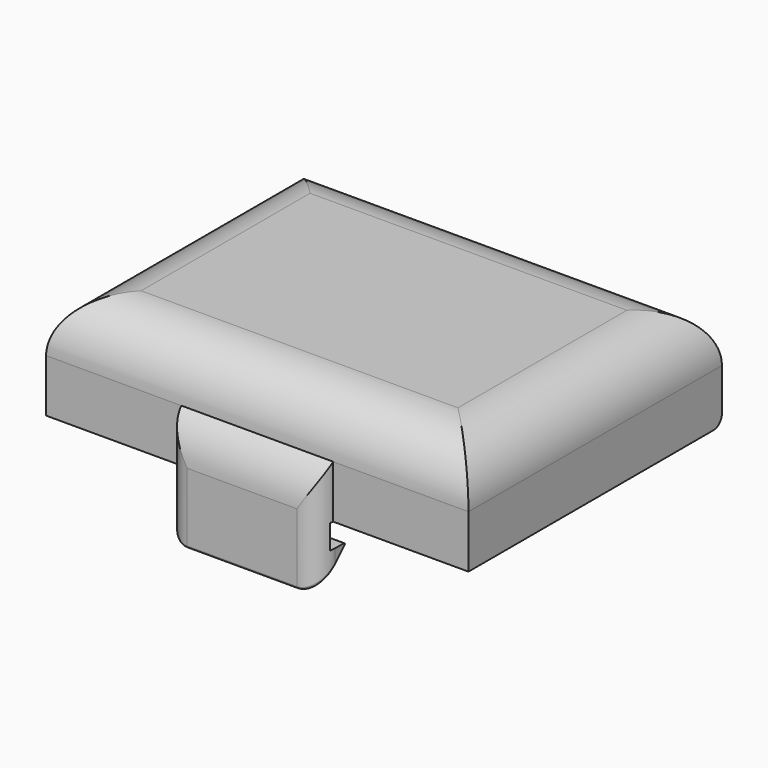
from build123d import *

# Parameters (mm, degrees)
F0_W          = 40
F0_H          = 30
F1_DEPTH      = 10
F2_R          = 5
F3_T          = -3
F4_W          = 27.6
F4_H          = 3
F5_DEPTH      = 3
F6_W          = 46.0305325687
F6_H          = 69.5610698313
F7_DEPTH      = 12.5
F8_R          = 0.55
F9_DEPTH      = 0.55
F10_R         = 0.54999
F11_R         = 1
F13_W         = 14.4
F13_H         = 12
F14_DEPTH     = 1.8
F16_DEPTH     = 25
F17_T4_DEPTH  = 20.8
F17_T9_DEPTH  = 20.8
F17_T14_DEPTH = 20.8
F17_T19_DEPTH = 20.8
F18_T1_DEPTH  = 29.6093727123
F19_R         = 0.2


# Not quite as in the source:
# - a fillet or chamfer that OpenCascade refuses, or shapes differently, is made with other operations: its cross-section is extruded or revolved along the edge and cut away or added
# - a fillet or chamfer is up to 0.001 mm smaller than in the source, because OpenCascade refuses the exact size


with BuildPart() as f1:
    # F0 (on Top) → F1 (new body)
    with BuildSketch(Plane.XY):
        Rectangle(F0_W, F0_H)
    extrude(amount=F1_DEPTH)

    # F2
    f2_edges = [f1.edges().sort_by_distance(p)[0] for p in [
        (20, 0, 10),
        (0, 15, 10),
        (-20, 0, 10),
        (0, -15, 10),
    ]]
    fillet(f2_edges, radius=F2_R)

    # F3
    f3_openings = [f1.faces().sort_by_distance(p)[0] for p in [
        (0, 0, 0),
    ]]
    offset(amount=F3_T, openings=f3_openings)

    # F4 (on Top) → F5 (join)
    with BuildSketch(Plane.XY):
        with Locations((0, 13.5)):
            Rectangle(F4_W, F4_H)
    extrude(amount=-F5_DEPTH)

    # F6 (on Top) → F7 (cut, symmetric)
    with BuildSketch(Plane.XY):
        with Locations((23.0152662843, -8.845419623)):
            Rectangle(F6_W, F6_H)
    extrude(amount=F7_DEPTH, both=True, mode=Mode.SUBTRACT)

    # F8 (on face) → F9 (join)
    with BuildSketch(Plane(origin=(-13.8, 0, 0), x_dir=(0, -1, 0), z_dir=(-1, 0, 0))):
        with Locations((-13.5, -1.5)):
            Circle(F8_R)
    extrude(amount=F9_DEPTH)

    # F10 (radius 0.55 in the source; OpenCascade refuses exactly that, so slightly less here)
    f10_edges = [f1.edges().sort_by_distance(p)[0] for p in [
        (-14.35, 14.05, -1.5),
    ]]
    fillet(f10_edges, radius=F10_R)

    # F11
    f11_edges = [f1.edges().sort_by_distance(p)[0] for p in [
        (-6.9, 15, -3),
        (-6.9, 12, -3),
        (-16.9, 15, 0),
        (-15.4, 12, 0),
    ]]
    fillet(f11_edges, radius=F11_R)

    # F12: F1 across plane


with BuildPart() as f1_1:
    add(f1.part)
    add(f1.part.mirror(Plane.YZ))

    # F13 (on face) → F14 (join, symmetric)
    with BuildSketch(Plane.XZ.offset(15)):
        with Locations((0, -1)):
            Rectangle(F13_W, F13_H)
    extrude(amount=F14_DEPTH, both=True)

    # F15 (on face) → F16 (cut)
    with BuildSketch(Plane(origin=(-7.2, 0, 0), x_dir=(0, -1, 0), z_dir=(-1, 0, 0))):
        Polygon((15.3, 0), (15, 0), (13.2, 0), (13.2, -7), (16.8, -7), (16.8, -5.8), (13.3, -2.3), (15.3, -2.3), align=None)
    extrude(amount=-F16_DEPTH, mode=Mode.SUBTRACT)

    # F17: fillet of radius 2 on 2 edges, made by hand


with BuildPart() as f17_tool2:
    # F17_s3 → F17_t4 (new body)
    with BuildSketch(Plane.XY.offset(10)):
        with BuildLine():
            ThreePointArc((-5.2, -16.8), (-6.6142135624, -16.2142135624), (-7.2, -14.8))
            Line((-7.2, -14.8), (-7.2, -16.8))
            Line((-7.2, -16.8), (-5.2, -16.8))
        make_face()
    extrude(amount=-F17_T4_DEPTH)

    split(bisect_by=Plane.XZ.offset(15), keep=Keep.TOP)


with BuildPart() as f1_2:
    add(f1_1.part)

    # F17_t1: cut F17_tool2
    add(f17_tool2.part, mode=Mode.SUBTRACT)


with BuildPart() as f17_tool7:
    # F17_s8 → F17_t9 (new body)
    with BuildSketch(Plane.XY.offset(10)):
        with BuildLine():
            ThreePointArc((-5.2, -16.8), (-6.6142135624, -16.2142135624), (-7.2, -14.8))
            Line((-7.2, -14.8), (-7.2, -16.8))
            Line((-7.2, -16.8), (-5.2, -16.8))
        make_face()
    extrude(amount=-F17_T9_DEPTH)

    split(bisect_by=Plane.XY, keep=Keep.BOTTOM)


with BuildPart() as f1_3:
    add(f1_2.part)

    # F17_t6: cut F17_tool7
    add(f17_tool7.part, mode=Mode.SUBTRACT)


with BuildPart() as f17_tool12:
    # F17_s13 → F17_t14 (new body)
    with BuildSketch(Plane.XY.offset(-10.8)):
        with BuildLine():
            ThreePointArc((5.2, -16.8), (6.6142135624, -16.2142135624), (7.2, -14.8))
            Line((7.2, -14.8), (7.2, -16.8))
            Line((7.2, -16.8), (5.2, -16.8))
        make_face()
    extrude(amount=F17_T14_DEPTH)

    split(bisect_by=Plane.XZ.offset(15), keep=Keep.TOP)


with BuildPart() as f1_4:
    add(f1_3.part)

    # F17_t11: cut F17_tool12
    add(f17_tool12.part, mode=Mode.SUBTRACT)


with BuildPart() as f17_tool17:
    # F17_s18 → F17_t19 (new body)
    with BuildSketch(Plane.XY.offset(-10.8)):
        with BuildLine():
            ThreePointArc((5.2, -16.8), (6.6142135624, -16.2142135624), (7.2, -14.8))
            Line((7.2, -14.8), (7.2, -16.8))
            Line((7.2, -16.8), (5.2, -16.8))
        make_face()
    extrude(amount=F17_T19_DEPTH)

    split(bisect_by=Plane.XY, keep=Keep.BOTTOM)


with BuildPart() as f1_5:
    add(f1_4.part)

    # F17_t16: cut F17_tool17
    add(f17_tool17.part, mode=Mode.SUBTRACT)

    # F18: fillet of radius 5 on 1 edges, made by hand

    # F18_s2 → F18_t1 (cut)
    with BuildSketch(Plane.YZ.offset(-14.8046863561)):
        with BuildLine():
            ThreePointArc((-16.8, 1.1581254575), (-16.3276925691, 3.2794458011), (-15, 5))
            Line((-15, 5), (-16.8, 5))
            Line((-16.8, 5), (-16.8, 1.1581254575))
        make_face()
    extrude(amount=F18_T1_DEPTH, mode=Mode.SUBTRACT)

    # F19
    f19_edges = [f1_5.edges().sort_by_distance(p)[0] for p in [
        (-7.2, -14.05, -3.05),
        (0, -13.3, -2.3),
        (7.2, -14.05, -3.05),
        (7.197495, -14.900063, -3.900063),
        (6.65083, -16.176624, -5.176624),
        (0, -16.8, -5.8),
        (-6.65083, -16.176624, -5.176624),
        (-7.197495, -14.900063, -3.900063),
    ]]
    fillet(f19_edges, radius=F19_R)


solid = f1_5.part
